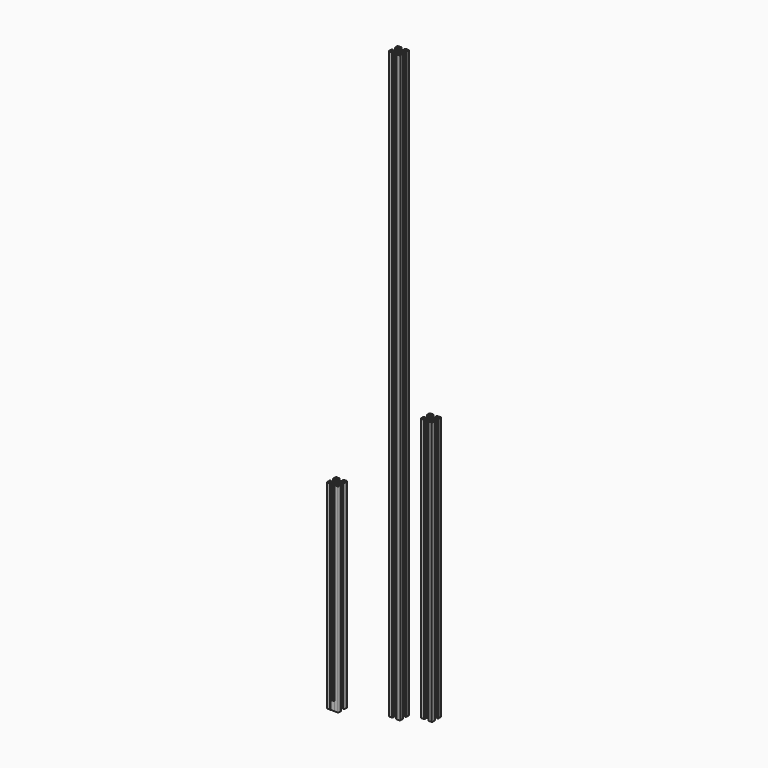
from build123d import *

# Parameters (mm, degrees)
F0_R     = 2.1
F1_DEPTH = 340
F2_DEPTH = 450
F3_DEPTH = 1000
F4_DEPTH = 15


# Not quite as in the source:
# - ends of sketch curves that miss each other by under 0.0002 mm in the source are joined


with BuildPart() as f1:
    # F0 (on Top) → F1 (new body)
    with BuildSketch(Plane.XY):
        with BuildLine():
            ThreePointArc((-10, 4.249657), (-9.9398646954, 3.9473367618), (-9.7686138571, 3.6910421429))
            Line((-9.7686138571, 3.6910421429), (-8.486151, 2.408579))
            ThreePointArc((-8.486151, 2.408579), (-8.272934613, 2.3633303292), (-8.1449896789, 2.5397919836))
            Line((-8.1449896789, 2.5397919836), (-8.14499, 3.6))
            Line((-8.14499, 3.6), (-5.028383, 3.6))
            Line((-5.028383, 3.6), (-3.4, 1.966096))
            Line((-3.4, 1.966096), (-3.4, 0.380897))
            Line((-3.4, 0.380897), (-3.019103, 0))
            Line((-3.019103, 0), (-3.4, -0.380897))
            Line((-3.4, -0.380897), (-3.4, -1.966096))
            Line((-3.4, -1.966096), (-5.028383, -3.6))
            Line((-5.028383, -3.6), (-8.14499, -3.6))
            Line((-8.14499, -3.6), (-8.14499, -2.539792))
            ThreePointArc((-8.14499, -2.539792), (-8.272934613, -2.3633303292), (-8.4861508562, -2.4085791438))
            Line((-8.4861508562, -2.4085791438), (-9.768614, -3.691042))
            ThreePointArc((-9.768614, -3.691042), (-9.9398646954, -3.9473367618), (-10, -4.249657))
            Line((-10, -4.249657), (-10, -8.580897))
            ThreePointArc((-10, -8.580897), (-9.5692782996, -9.5571257282), (-8.5985019868, -9.9999997949))
            Line((-8.5985019868, -9.9999997949), (-4.042831, -10))
            ThreePointArc((-4.042831, -10), (-3.7366842541, -9.939103626), (-3.4771455751, -9.7656854249))
            Line((-3.4771455751, -9.7656854249), (-2.373223, -8.661763))
            ThreePointArc((-2.373223, -8.661763), (-2.3190301169, -8.3893151419), (-2.55, -8.234986))
            Line((-2.55, -8.234986), (-3.2809961147, -8.234986))
            Line((-3.2809961147, -8.234986), (-3.6, -8.234986))
            Line((-3.6, -8.234986), (-3.6, -5.034986))
            Line((-3.6, -5.034986), (-2.005406, -3.434986))
            Line((-2.005406, -3.434986), (-0.3, -3.434986))
            Line((-0.3, -3.434986), (0, -3.175033))
            Line((0, -3.175033), (0.3, -3.434986))
            Line((0.3, -3.434986), (2.005406, -3.434986))
            Line((2.005406, -3.434986), (3.6, -5.034986))
            Line((3.6, -5.034986), (3.6, -8.234986))
            Line((3.6, -8.234986), (2.7389244642, -8.234986))
            Line((2.7389244642, -8.234986), (2.55, -8.234986))
            ThreePointArc((2.55, -8.234986), (2.3190301169, -8.3893151419), (2.3732233047, -8.6617626953))
            Line((2.3732233047, -8.6617626953), (3.477146, -9.7656854249))
            ThreePointArc((3.477146, -9.7656854249), (3.7366842541, -9.939103626), (4.042831, -10))
            Line((4.042831, -10), (8.598502, -10))
            ThreePointArc((8.598502, -10), (9.5692782996, -9.5571257282), (10.000000494, -8.5808970257))
            Line((10.000000494, -8.5808970257), (10, -4.249657))
            ThreePointArc((10, -4.249657), (9.9398646954, -3.9473367618), (9.7686138571, -3.6910421429))
            Line((9.7686138571, -3.6910421429), (8.486151, -2.408579))
            ThreePointArc((8.486151, -2.408579), (8.272934613, -2.3633303292), (8.1449896789, -2.5397919836))
            Line((8.1449896789, -2.5397919836), (8.14499, -3.6))
            Line((8.14499, -3.6), (5.028383, -3.6))
            Line((5.028383, -3.6), (3.4, -1.966096))
            Line((3.4, -1.966096), (3.4, -0.380897))
            Line((3.4, -0.380897), (3.019103, 0))
            Line((3.019103, 0), (3.4, 0.380897))
            Line((3.4, 0.380897), (3.4, 1.966096))
            Line((3.4, 1.966096), (5.028383, 3.6))
            Line((5.028383, 3.6), (8.14499, 3.6))
            Line((8.14499, 3.6), (8.14499, 2.539792))
            ThreePointArc((8.14499, 2.539792), (8.272934613, 2.3633303292), (8.4861508562, 2.4085791438))
            Line((8.4861508562, 2.4085791438), (9.768614, 3.691042))
            ThreePointArc((9.768614, 3.691042), (9.9398646954, 3.9473367618), (10, 4.249657))
            Line((10, 4.249657), (10, 8.580897))
            ThreePointArc((10, 8.580897), (9.5692782996, 9.5571257282), (8.5985019868, 9.9999997949))
            Line((8.5985019868, 9.9999997949), (4.042831, 10))
            ThreePointArc((4.042831, 10), (3.7366842541, 9.939103626), (3.4771455751, 9.7656854249))
            Line((3.4771455751, 9.7656854249), (2.373223, 8.661763))
            ThreePointArc((2.373223, 8.661763), (2.3190301169, 8.3893151419), (2.55, 8.234986))
            Line((2.55, 8.234986), (3.6, 8.234986))
            Line((3.6, 8.234986), (3.6, 5.034986))
            Line((3.6, 5.034986), (2.005406, 3.434986))
            Line((2.005406, 3.434986), (0.3, 3.434986))
            Line((0.3, 3.434986), (0, 3.175033))
            Line((0, 3.175033), (-0.3, 3.434986))
            Line((-0.3, 3.434986), (-2.005406, 3.434986))
            Line((-2.005406, 3.434986), (-3.6, 5.034986))
            Line((-3.6, 5.034986), (-3.6, 8.234986))
            Line((-3.6, 8.234986), (-2.55, 8.234986))
            ThreePointArc((-2.55, 8.234986), (-2.3190301169, 8.3893151419), (-2.3732233047, 8.6617626953))
            Line((-2.3732233047, 8.6617626953), (-3.477146, 9.765685))
            ThreePointArc((-3.477146, 9.765685), (-3.7366842541, 9.939103626), (-4.042831, 10))
            Line((-4.042831, 10), (-8.598502, 10))
            ThreePointArc((-8.598502, 10), (-9.5692782996, 9.5571257282), (-10.000000494, 8.5808970257))
            Line((-10.000000494, 8.5808970257), (-10, 4.249657))
        make_face()
        with BuildLine():
            Line((-8.8, -8.380897), (-8.8, -5.380897))
            ThreePointArc((-8.8, -5.380897), (-8.715797611, -5.0044798769), (-8.388737989, -4.8000000672))
            Line((-8.388737989, -4.8000000672), (-5.388738, -4.8))
            ThreePointArc((-5.388738, -4.8), (-4.9405856758, -4.9345894318), (-4.7999996015, -5.3808970733))
            Line((-4.7999996015, -5.3808970733), (-4.8, -8.380897))
            ThreePointArc((-4.8, -8.380897), (-5.0082634718, -8.7203834023), (-5.3985019161, -8.7999996031))
            Line((-5.3985019161, -8.7999996031), (-8.398502, -8.8))
            ThreePointArc((-8.398502, -8.8), (-8.6662842471, -8.6546658673), (-8.8, -8.380897))
        make_face(mode=Mode.SUBTRACT)
        with BuildLine():
            ThreePointArc((4.7999996015, -5.3808970733), (4.9405856758, -4.9345894318), (5.3887380594, -4.7999996994))
            Line((5.3887380594, -4.7999996994), (8.388738, -4.8))
            ThreePointArc((8.388738, -4.8), (8.715797611, -5.0044798769), (8.8000003179, -5.3808970565))
            Line((8.8000003179, -5.3808970565), (8.8, -8.380897))
            ThreePointArc((8.8, -8.380897), (8.6662842471, -8.6546658673), (8.3985020208, -8.8000001098))
            Line((8.3985020208, -8.8000001098), (5.398502, -8.8))
            ThreePointArc((5.398502, -8.8), (5.0082634718, -8.7203834023), (4.7999997135, -8.3808970406))
            Line((4.7999997135, -8.3808970406), (4.7999996015, -5.3808970733))
        make_face(mode=Mode.SUBTRACT)
        Circle(F0_R, mode=Mode.SUBTRACT)
        with BuildLine():
            ThreePointArc((-4.7999996015, 5.3808970733), (-4.9405856758, 4.9345894318), (-5.3887380594, 4.7999996994))
            Line((-5.3887380594, 4.7999996994), (-8.388738, 4.8))
            ThreePointArc((-8.388738, 4.8), (-8.715797611, 5.0044798769), (-8.8000003179, 5.3808970565))
            Line((-8.8000003179, 5.3808970565), (-8.8, 8.380897))
            ThreePointArc((-8.8, 8.380897), (-8.6662842471, 8.6546658673), (-8.3985020208, 8.8000001098))
            Line((-8.3985020208, 8.8000001098), (-5.398502, 8.8))
            ThreePointArc((-5.398502, 8.8), (-5.0082634718, 8.7203834023), (-4.7999997135, 8.3808970406))
            Line((-4.7999997135, 8.3808970406), (-4.7999996015, 5.3808970733))
        make_face(mode=Mode.SUBTRACT)
        with BuildLine():
            Line((8.8, 8.380897), (8.8, 5.380897))
            ThreePointArc((8.8, 5.380897), (8.715797611, 5.0044798769), (8.388737989, 4.8000000672))
            Line((8.388737989, 4.8000000672), (5.388738, 4.8))
            ThreePointArc((5.388738, 4.8), (4.9405856758, 4.9345894318), (4.7999996015, 5.3808970733))
            Line((4.7999996015, 5.3808970733), (4.8, 8.380897))
            ThreePointArc((4.8, 8.380897), (5.0082634718, 8.7203834023), (5.3985019161, 8.7999996031))
            Line((5.3985019161, 8.7999996031), (8.398502, 8.8))
            ThreePointArc((8.398502, 8.8), (8.6662842471, 8.6546658673), (8.8, 8.380897))
        make_face(mode=Mode.SUBTRACT)
    extrude(amount=F1_DEPTH)


with BuildPart() as f2:
    # F0 (on Top) → F2 (new body)
    with BuildSketch(Plane.XY):
        with BuildLine():
            ThreePointArc((104.7369111792, 61.2872370619), (104.7970464838, 60.9849168237), (104.9682973221, 60.7286222047))
            Line((104.9682973221, 60.7286222047), (106.2507601792, 59.4461590619))
            ThreePointArc((106.2507601792, 59.4461590619), (106.4639765663, 59.4009103911), (106.5919215003, 59.5773720455))
            Line((106.5919215003, 59.5773720455), (106.5919211792, 60.6375800619))
            Line((106.5919211792, 60.6375800619), (109.7085281792, 60.6375800619))
            Line((109.7085281792, 60.6375800619), (111.3369111792, 59.0036760619))
            Line((111.3369111792, 59.0036760619), (111.3369111792, 57.4184770619))
            Line((111.3369111792, 57.4184770619), (111.7178081792, 57.0375800619))
            Line((111.7178081792, 57.0375800619), (111.3369111792, 56.6566830619))
            Line((111.3369111792, 56.6566830619), (111.3369111792, 55.0714840619))
            Line((111.3369111792, 55.0714840619), (109.7085281792, 53.4375800619))
            Line((109.7085281792, 53.4375800619), (106.5919211792, 53.4375800619))
            Line((106.5919211792, 53.4375800619), (106.5919211792, 54.4977880619))
            ThreePointArc((106.5919211792, 54.4977880619), (106.4639765663, 54.6742497327), (106.250760323, 54.6290009181))
            Line((106.250760323, 54.6290009181), (104.9682971792, 53.3465380619))
            ThreePointArc((104.9682971792, 53.3465380619), (104.7970464838, 53.0902433001), (104.7369111792, 52.7879230619))
            Line((104.7369111792, 52.7879230619), (104.7369111792, 48.4566830619))
            ThreePointArc((104.7369111792, 48.4566830619), (105.1676328796, 47.4804543337), (106.1384091924, 47.037580267))
            Line((106.1384091924, 47.037580267), (110.6940801792, 47.0375800619))
            ThreePointArc((110.6940801792, 47.0375800619), (111.0002269251, 47.0984764359), (111.2597656042, 47.2718946369))
            Line((111.2597656042, 47.2718946369), (112.3636881792, 48.3758170619))
            ThreePointArc((112.3636881792, 48.3758170619), (112.4178810623, 48.64826492), (112.1869111792, 48.8025940619))
            Line((112.1869111792, 48.8025940619), (111.1369111792, 48.8025940619))
            Line((111.1369111792, 48.8025940619), (111.1369111792, 52.0025940619))
            Line((111.1369111792, 52.0025940619), (112.7315051792, 53.6025940619))
            Line((112.7315051792, 53.6025940619), (114.4369111792, 53.6025940619))
            Line((114.4369111792, 53.6025940619), (114.7369111792, 53.8625470619))
            Line((114.7369111792, 53.8625470619), (115.0369111792, 53.6025940619))
            Line((115.0369111792, 53.6025940619), (116.7423171792, 53.6025940619))
            Line((116.7423171792, 53.6025940619), (118.3369111792, 52.0025940619))
            Line((118.3369111792, 52.0025940619), (118.3369111792, 48.8025940619))
            Line((118.3369111792, 48.8025940619), (117.2869111792, 48.8025940619))
            ThreePointArc((117.2869111792, 48.8025940619), (117.0559412961, 48.64826492), (117.1101344839, 48.3758173666))
            Line((117.1101344839, 48.3758173666), (118.2140571792, 47.2718950619))
            ThreePointArc((118.2140571792, 47.2718950619), (118.4735954333, 47.0984764359), (118.7797421792, 47.0375800619))
            Line((118.7797421792, 47.0375800619), (123.3354131792, 47.0375800619))
            ThreePointArc((123.3354131792, 47.0375800619), (124.3061894788, 47.4804543337), (124.7369116732, 48.4566830362))
            Line((124.7369116732, 48.4566830362), (124.7369111792, 52.7879230619))
            ThreePointArc((124.7369111792, 52.7879230619), (124.6767758746, 53.0902433001), (124.5055250364, 53.346537919))
            Line((124.5055250364, 53.346537919), (123.2230621792, 54.6290010619))
            ThreePointArc((123.2230621792, 54.6290010619), (123.0098457922, 54.6742497327), (122.8819008581, 54.4977880783))
            Line((122.8819008581, 54.4977880783), (122.8819011792, 53.4375800619))
            Line((122.8819011792, 53.4375800619), (119.7652941792, 53.4375800619))
            Line((119.7652941792, 53.4375800619), (118.1369111792, 55.0714840619))
            Line((118.1369111792, 55.0714840619), (118.1369111792, 56.6566830619))
            Line((118.1369111792, 56.6566830619), (117.7560141792, 57.0375800619))
            Line((117.7560141792, 57.0375800619), (118.1369111792, 57.4184770619))
            Line((118.1369111792, 57.4184770619), (118.1369111792, 59.0036760619))
            Line((118.1369111792, 59.0036760619), (119.7652941792, 60.6375800619))
            Line((119.7652941792, 60.6375800619), (122.8819011792, 60.6375800619))
            Line((122.8819011792, 60.6375800619), (122.8819011792, 59.5773720619))
            ThreePointArc((122.8819011792, 59.5773720619), (123.0098457922, 59.4009103911), (123.2230620354, 59.4461592056))
            Line((123.2230620354, 59.4461592056), (124.5055251792, 60.7286220619))
            ThreePointArc((124.5055251792, 60.7286220619), (124.6767758746, 60.9849168237), (124.7369111792, 61.2872370619))
            Line((124.7369111792, 61.2872370619), (124.7369111792, 65.6184770619))
            ThreePointArc((124.7369111792, 65.6184770619), (124.3061894788, 66.5947057901), (123.335413166, 67.0375798568))
            Line((123.335413166, 67.0375798568), (118.7797421792, 67.0375800619))
            ThreePointArc((118.7797421792, 67.0375800619), (118.4735954333, 66.9766836879), (118.2140567543, 66.8032654868))
            Line((118.2140567543, 66.8032654868), (117.1101341792, 65.6993430619))
            ThreePointArc((117.1101341792, 65.6993430619), (117.0559412961, 65.4268952038), (117.2869111792, 65.2725660619))
            Line((117.2869111792, 65.2725660619), (118.3369111792, 65.2725660619))
            Line((118.3369111792, 65.2725660619), (118.3369111792, 62.0725660619))
            Line((118.3369111792, 62.0725660619), (116.7423171792, 60.4725660619))
            Line((116.7423171792, 60.4725660619), (115.0369111792, 60.4725660619))
            Line((115.0369111792, 60.4725660619), (114.7369111792, 60.2126130619))
            Line((114.7369111792, 60.2126130619), (114.4369111792, 60.4725660619))
            Line((114.4369111792, 60.4725660619), (112.7315051792, 60.4725660619))
            Line((112.7315051792, 60.4725660619), (111.1369111792, 62.0725660619))
            Line((111.1369111792, 62.0725660619), (111.1369111792, 65.2725660619))
            Line((111.1369111792, 65.2725660619), (112.1869111792, 65.2725660619))
            ThreePointArc((112.1869111792, 65.2725660619), (112.4178810623, 65.4268952038), (112.3636878745, 65.6993427572))
            Line((112.3636878745, 65.6993427572), (111.2597651792, 66.8032650619))
            ThreePointArc((111.2597651792, 66.8032650619), (111.0002269251, 66.9766836879), (110.6940801792, 67.0375800619))
            Line((110.6940801792, 67.0375800619), (106.1384091792, 67.0375800619))
            ThreePointArc((106.1384091792, 67.0375800619), (105.1676328796, 66.5947057901), (104.7369106852, 65.6184770875))
            Line((104.7369106852, 65.6184770875), (104.7369111792, 61.2872370619))
        make_face()
        with BuildLine():
            Line((105.9369111792, 48.6566830619), (105.9369111792, 51.6566830619))
            ThreePointArc((105.9369111792, 51.6566830619), (106.0211135682, 52.033100185), (106.3481731902, 52.2375799947))
            Line((106.3481731902, 52.2375799947), (109.3481731792, 52.2375800619))
            ThreePointArc((109.3481731792, 52.2375800619), (109.7963255034, 52.10299063), (109.9369115778, 51.6566829886))
            Line((109.9369115778, 51.6566829886), (109.9369111792, 48.6566830619))
            ThreePointArc((109.9369111792, 48.6566830619), (109.7286477074, 48.3171966596), (109.3384092631, 48.2375804588))
            Line((109.3384092631, 48.2375804588), (106.3384091792, 48.2375800619))
            ThreePointArc((106.3384091792, 48.2375800619), (106.0706269321, 48.3829141945), (105.9369111792, 48.6566830619))
        make_face(mode=Mode.SUBTRACT)
        with BuildLine():
            ThreePointArc((119.5369107807, 51.6566829886), (119.677496855, 52.10299063), (120.1256492386, 52.2375803625))
            Line((120.1256492386, 52.2375803625), (123.1256491792, 52.2375800619))
            ThreePointArc((123.1256491792, 52.2375800619), (123.4527087903, 52.033100185), (123.5369114971, 51.6566830054))
            Line((123.5369114971, 51.6566830054), (123.5369111792, 48.6566830619))
            ThreePointArc((123.5369111792, 48.6566830619), (123.4031954263, 48.3829141945), (123.1354132001, 48.2375799521))
            Line((123.1354132001, 48.2375799521), (120.1354131792, 48.2375800619))
            ThreePointArc((120.1354131792, 48.2375800619), (119.745174651, 48.3171966596), (119.5369108927, 48.6566830213))
            Line((119.5369108927, 48.6566830213), (119.5369107807, 51.6566829886))
        make_face(mode=Mode.SUBTRACT)
        with Locations((114.7369111792, 57.0375800619)):
            Circle(F0_R, mode=Mode.SUBTRACT)
        with BuildLine():
            ThreePointArc((109.9369115778, 62.4184771351), (109.7963255034, 61.9721694937), (109.3481731198, 61.8375797612))
            Line((109.3481731198, 61.8375797612), (106.3481731792, 61.8375800619))
            ThreePointArc((106.3481731792, 61.8375800619), (106.0211135682, 62.0420599388), (105.9369108613, 62.4184771184))
            Line((105.9369108613, 62.4184771184), (105.9369111792, 65.4184770619))
            ThreePointArc((105.9369111792, 65.4184770619), (106.0706269321, 65.6922459292), (106.3384091584, 65.8375801717))
            Line((106.3384091584, 65.8375801717), (109.3384091792, 65.8375800619))
            ThreePointArc((109.3384091792, 65.8375800619), (109.7286477074, 65.7579634642), (109.9369114657, 65.4184771024))
            Line((109.9369114657, 65.4184771024), (109.9369115778, 62.4184771351))
        make_face(mode=Mode.SUBTRACT)
        with BuildLine():
            Line((123.5369111792, 65.4184770619), (123.5369111792, 62.4184770619))
            ThreePointArc((123.5369111792, 62.4184770619), (123.4527087903, 62.0420599388), (123.1256491682, 61.8375801291))
            Line((123.1256491682, 61.8375801291), (120.1256491792, 61.8375800619))
            ThreePointArc((120.1256491792, 61.8375800619), (119.677496855, 61.9721694937), (119.5369107807, 62.4184771351))
            Line((119.5369107807, 62.4184771351), (119.5369111792, 65.4184770619))
            ThreePointArc((119.5369111792, 65.4184770619), (119.745174651, 65.7579634642), (120.1354130953, 65.837579665))
            Line((120.1354130953, 65.837579665), (123.1354131792, 65.8375800619))
            ThreePointArc((123.1354131792, 65.8375800619), (123.4031954263, 65.6922459292), (123.5369111792, 65.4184770619))
        make_face(mode=Mode.SUBTRACT)
    extrude(amount=F2_DEPTH)


with BuildPart() as f3:
    # F0 (on Top) → F3 (new body)
    with BuildSketch(Plane.XY):
        with BuildLine():
            ThreePointArc((68.5801450626, 37.9286163587), (68.6402803672, 37.6262961204), (68.8115312055, 37.3700015015))
            Line((68.8115312055, 37.3700015015), (70.0939940626, 36.0875383587))
            ThreePointArc((70.0939940626, 36.0875383587), (70.3072104496, 36.0422896879), (70.4351553837, 36.2187513422))
            Line((70.4351553837, 36.2187513422), (70.4351550626, 37.2789593587))
            Line((70.4351550626, 37.2789593587), (73.5517620626, 37.2789593587))
            Line((73.5517620626, 37.2789593587), (75.1801450626, 35.6450553587))
            Line((75.1801450626, 35.6450553587), (75.1801450626, 34.0598563587))
            Line((75.1801450626, 34.0598563587), (75.5610420626, 33.6789593587))
            Line((75.5610420626, 33.6789593587), (75.1801450626, 33.2980623587))
            Line((75.1801450626, 33.2980623587), (75.1801450626, 31.7128633587))
            Line((75.1801450626, 31.7128633587), (73.5517620626, 30.0789593587))
            Line((73.5517620626, 30.0789593587), (70.4351550626, 30.0789593587))
            Line((70.4351550626, 30.0789593587), (70.4351550626, 31.1391673587))
            ThreePointArc((70.4351550626, 31.1391673587), (70.3072104496, 31.3156290294), (70.0939942064, 31.2703802149))
            Line((70.0939942064, 31.2703802149), (68.8115310626, 29.9879173587))
            ThreePointArc((68.8115310626, 29.9879173587), (68.6402803672, 29.7316225969), (68.5801450626, 29.4293023587))
            Line((68.5801450626, 29.4293023587), (68.5801450626, 25.0980623587))
            ThreePointArc((68.5801450626, 25.0980623587), (69.010866763, 24.1218336304), (69.9816430758, 23.6789595637))
            Line((69.9816430758, 23.6789595637), (74.5373140626, 23.6789593587))
            ThreePointArc((74.5373140626, 23.6789593587), (74.8434608085, 23.7398557326), (75.1029994875, 23.9132739337))
            Line((75.1029994875, 23.9132739337), (76.2069220626, 25.0171963587))
            ThreePointArc((76.2069220626, 25.0171963587), (76.2611149457, 25.2896442167), (76.0301450626, 25.4439733587))
            Line((76.0301450626, 25.4439733587), (74.9801450626, 25.4439733587))
            Line((74.9801450626, 25.4439733587), (74.9801450626, 28.6439733587))
            Line((74.9801450626, 28.6439733587), (76.5747390626, 30.2439733587))
            Line((76.5747390626, 30.2439733587), (78.2801450626, 30.2439733587))
            Line((78.2801450626, 30.2439733587), (78.5801450626, 30.5039263587))
            Line((78.5801450626, 30.5039263587), (78.8801450626, 30.2439733587))
            Line((78.8801450626, 30.2439733587), (80.5855510626, 30.2439733587))
            Line((80.5855510626, 30.2439733587), (82.1801450626, 28.6439733587))
            Line((82.1801450626, 28.6439733587), (82.1801450626, 25.4439733587))
            Line((82.1801450626, 25.4439733587), (81.1301450626, 25.4439733587))
            ThreePointArc((81.1301450626, 25.4439733587), (80.8991751795, 25.2896442167), (80.9533683673, 25.0171966634))
            Line((80.9533683673, 25.0171966634), (82.0572910626, 23.9132743587))
            ThreePointArc((82.0572910626, 23.9132743587), (82.3168293167, 23.7398557326), (82.6229760626, 23.6789593587))
            Line((82.6229760626, 23.6789593587), (87.1786470626, 23.6789593587))
            ThreePointArc((87.1786470626, 23.6789593587), (88.1494233622, 24.1218336304), (88.5801455566, 25.098062333))
            Line((88.5801455566, 25.098062333), (88.5801450626, 29.4293023587))
            ThreePointArc((88.5801450626, 29.4293023587), (88.520009758, 29.7316225969), (88.3487589197, 29.9879172158))
            Line((88.3487589197, 29.9879172158), (87.0662960626, 31.2703803587))
            ThreePointArc((87.0662960626, 31.2703803587), (86.8530796755, 31.3156290294), (86.7251347415, 31.1391673751))
            Line((86.7251347415, 31.1391673751), (86.7251350626, 30.0789593587))
            Line((86.7251350626, 30.0789593587), (83.6085280626, 30.0789593587))
            Line((83.6085280626, 30.0789593587), (81.9801450626, 31.7128633587))
            Line((81.9801450626, 31.7128633587), (81.9801450626, 33.2980623587))
            Line((81.9801450626, 33.2980623587), (81.5992480626, 33.6789593587))
            Line((81.5992480626, 33.6789593587), (81.9801450626, 34.0598563587))
            Line((81.9801450626, 34.0598563587), (81.9801450626, 35.6450553587))
            Line((81.9801450626, 35.6450553587), (83.6085280626, 37.2789593587))
            Line((83.6085280626, 37.2789593587), (86.7251350626, 37.2789593587))
            Line((86.7251350626, 37.2789593587), (86.7251350626, 36.2187513587))
            ThreePointArc((86.7251350626, 36.2187513587), (86.8530796755, 36.0422896879), (87.0662959188, 36.0875385024))
            Line((87.0662959188, 36.0875385024), (88.3487590626, 37.3700013587))
            ThreePointArc((88.3487590626, 37.3700013587), (88.520009758, 37.6262961204), (88.5801450626, 37.9286163587))
            Line((88.5801450626, 37.9286163587), (88.5801450626, 42.2598563587))
            ThreePointArc((88.5801450626, 42.2598563587), (88.1494233622, 43.2360850869), (87.1786470494, 43.6789591536))
            Line((87.1786470494, 43.6789591536), (82.6229760626, 43.6789593587))
            ThreePointArc((82.6229760626, 43.6789593587), (82.3168293167, 43.6180629847), (82.0572906376, 43.4446447836))
            Line((82.0572906376, 43.4446447836), (80.9533680626, 42.3407223587))
            ThreePointArc((80.9533680626, 42.3407223587), (80.8991751795, 42.0682745006), (81.1301450626, 41.9139453587))
            Line((81.1301450626, 41.9139453587), (82.1801450626, 41.9139453587))
            Line((82.1801450626, 41.9139453587), (82.1801450626, 38.7139453587))
            Line((82.1801450626, 38.7139453587), (80.5855510626, 37.1139453587))
            Line((80.5855510626, 37.1139453587), (78.8801450626, 37.1139453587))
            Line((78.8801450626, 37.1139453587), (78.5801450626, 36.8539923587))
            Line((78.5801450626, 36.8539923587), (78.2801450626, 37.1139453587))
            Line((78.2801450626, 37.1139453587), (76.5747390626, 37.1139453587))
            Line((76.5747390626, 37.1139453587), (74.9801450626, 38.7139453587))
            Line((74.9801450626, 38.7139453587), (74.9801450626, 41.9139453587))
            Line((74.9801450626, 41.9139453587), (76.0301450626, 41.9139453587))
            ThreePointArc((76.0301450626, 41.9139453587), (76.2611149457, 42.0682745006), (76.2069217579, 42.340722054))
            Line((76.2069217579, 42.340722054), (75.1029990626, 43.4446443587))
            ThreePointArc((75.1029990626, 43.4446443587), (74.8434608085, 43.6180629847), (74.5373140626, 43.6789593587))
            Line((74.5373140626, 43.6789593587), (69.9816430626, 43.6789593587))
            ThreePointArc((69.9816430626, 43.6789593587), (69.010866763, 43.2360850869), (68.5801445686, 42.2598563843))
            Line((68.5801445686, 42.2598563843), (68.5801450626, 37.9286163587))
        make_face()
        with BuildLine():
            Line((69.7801450626, 25.2980623587), (69.7801450626, 28.2980623587))
            ThreePointArc((69.7801450626, 28.2980623587), (69.8643474515, 28.6744794818), (70.1914070736, 28.8789592914))
            Line((70.1914070736, 28.8789592914), (73.1914070626, 28.8789593587))
            ThreePointArc((73.1914070626, 28.8789593587), (73.6395593868, 28.7443699268), (73.7801454611, 28.2980622854))
            Line((73.7801454611, 28.2980622854), (73.7801450626, 25.2980623587))
            ThreePointArc((73.7801450626, 25.2980623587), (73.5718815908, 24.9585759564), (73.1816431465, 24.8789597556))
            Line((73.1816431465, 24.8789597556), (70.1816430626, 24.8789593587))
            ThreePointArc((70.1816430626, 24.8789593587), (69.9138608155, 25.0242934913), (69.7801450626, 25.2980623587))
        make_face(mode=Mode.SUBTRACT)
        with BuildLine():
            ThreePointArc((83.3801446641, 28.2980622854), (83.5207307384, 28.7443699268), (83.968883122, 28.8789596593))
            Line((83.968883122, 28.8789596593), (86.9688830626, 28.8789593587))
            ThreePointArc((86.9688830626, 28.8789593587), (87.2959426736, 28.6744794818), (87.3801453805, 28.2980623021))
            Line((87.3801453805, 28.2980623021), (87.3801450626, 25.2980623587))
            ThreePointArc((87.3801450626, 25.2980623587), (87.2464293097, 25.0242934913), (86.9786470834, 24.8789592489))
            Line((86.9786470834, 24.8789592489), (83.9786470626, 24.8789593587))
            ThreePointArc((83.9786470626, 24.8789593587), (83.5884085344, 24.9585759564), (83.3801447761, 25.2980623181))
            Line((83.3801447761, 25.2980623181), (83.3801446641, 28.2980622854))
        make_face(mode=Mode.SUBTRACT)
        with Locations((78.5801450626, 33.6789593587)):
            Circle(F0_R, mode=Mode.SUBTRACT)
        with BuildLine():
            ThreePointArc((73.7801454611, 39.0598564319), (73.6395593868, 38.6135487905), (73.1914070032, 38.478959058))
            Line((73.1914070032, 38.478959058), (70.1914070626, 38.4789593587))
            ThreePointArc((70.1914070626, 38.4789593587), (69.8643474515, 38.6834392355), (69.7801447447, 39.0598564152))
            Line((69.7801447447, 39.0598564152), (69.7801450626, 42.0598563587))
            ThreePointArc((69.7801450626, 42.0598563587), (69.9138608155, 42.333625226), (70.1816430417, 42.4789594684))
            Line((70.1816430417, 42.4789594684), (73.1816430626, 42.4789593587))
            ThreePointArc((73.1816430626, 42.4789593587), (73.5718815908, 42.3993427609), (73.7801453491, 42.0598563992))
            Line((73.7801453491, 42.0598563992), (73.7801454611, 39.0598564319))
        make_face(mode=Mode.SUBTRACT)
        with BuildLine():
            Line((87.3801450626, 42.0598563587), (87.3801450626, 39.0598563587))
            ThreePointArc((87.3801450626, 39.0598563587), (87.2959426736, 38.6834392355), (86.9688830516, 38.4789594259))
            Line((86.9688830516, 38.4789594259), (83.9688830626, 38.4789593587))
            ThreePointArc((83.9688830626, 38.4789593587), (83.5207307384, 38.6135487905), (83.3801446641, 39.0598564319))
            Line((83.3801446641, 39.0598564319), (83.3801450626, 42.0598563587))
            ThreePointArc((83.3801450626, 42.0598563587), (83.5884085344, 42.3993427609), (83.9786469787, 42.4789589617))
            Line((83.9786469787, 42.4789589617), (86.9786470626, 42.4789593587))
            ThreePointArc((86.9786470626, 42.4789593587), (87.2464293097, 42.333625226), (87.3801450626, 42.0598563587))
        make_face(mode=Mode.SUBTRACT)
    extrude(amount=F3_DEPTH)


with BuildPart() as f4:
    # F0 (on Top) → F4 (new body)
    with BuildSketch(Plane.XY):
        with BuildLine():
            Line((-2.373223, -8.661763), (-3.477146, -9.765685))
            Line((-3.477146, -9.765685), (3.477146, -9.7656854249))
            Line((3.477146, -9.7656854249), (2.373223, -8.6617634249))
            ThreePointArc((2.373223, -8.6617634249), (2.3190301169, -8.3893151419), (2.55, -8.234986))
            Line((2.55, -8.234986), (2.7389244642, -8.234986))
            Line((2.7389244642, -8.234986), (2.7389244642, -7.4637952166))
            Line((2.7389244642, -7.4637952166), (-3.4519615293, -7.4432836737))
            Line((-3.4519615293, -7.4432836737), (-3.4479278591, -8.0056138611))
            Line((-3.4479278591, -8.0056138611), (-3.2809961147, -8.234986))
            Line((-3.2809961147, -8.234986), (-2.55, -8.234986))
            ThreePointArc((-2.55, -8.234986), (-2.3190301169, -8.3893151419), (-2.373223, -8.661763))
        make_face()
    extrude(amount=F4_DEPTH)


solid = Compound([f1.part, f2.part, f3.part, f4.part])
